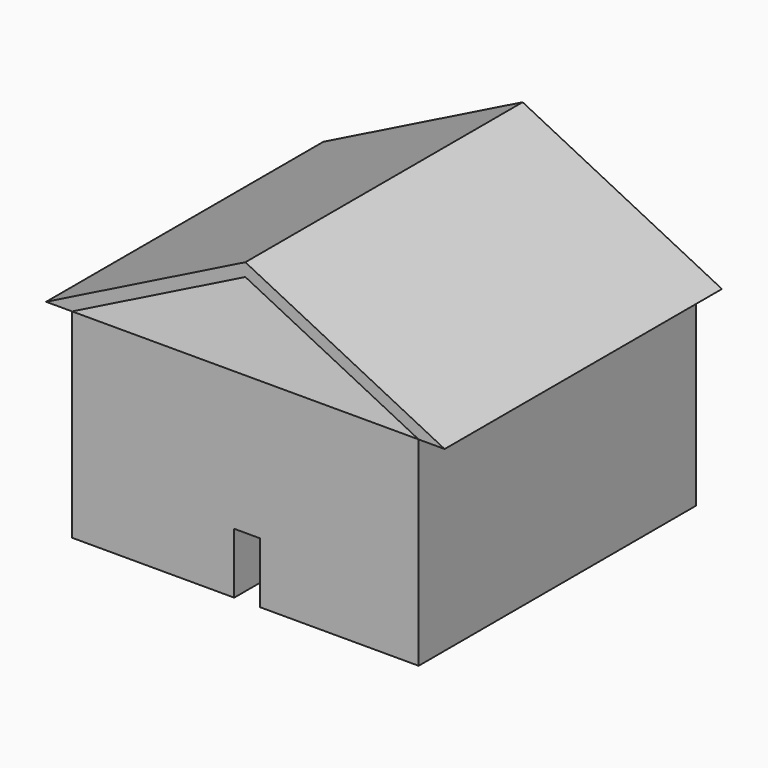
from build123d import *

# Parameters (mm, degrees)
F1_DEPTH = 6096


# Not quite as in the source:
# - the program builds the solid bodies; features that only make, move or delete a surface that nothing else refers to are left out


with BuildPart() as f1:
    # F0 (on Front) → F1 (new body, symmetric)
    with BuildSketch(Plane.XZ):
        Polygon((-7010.4, 0), (-6096, 0), (0, 3048), (0, 3505.2), align=None)
        Polygon((0, 3048), (6096, 0), (7010.4, 0), (0, 3505.2), align=None)
    extrude(amount=F1_DEPTH, both=True)


with BuildPart() as f1b:
    # F0 (on Front) → F1, piece 2 (new body, symmetric)
    with BuildSketch(Plane.XZ):
        Polygon((0, -4876.8), (0, 0), (-6096, 0), (-6096, -7010.4), (-391.4279341698, -7010.4), (-391.4279341698, -4876.8), align=None)
        Polygon((6096, 0), (0, 0), (0, -4876.8), (522.9720658302, -4876.8), (522.9720658302, -7010.4), (6096, -7010.4), align=None)
    extrude(amount=F1_DEPTH, both=True)


solid = Compound([f1.part, f1b.part])
